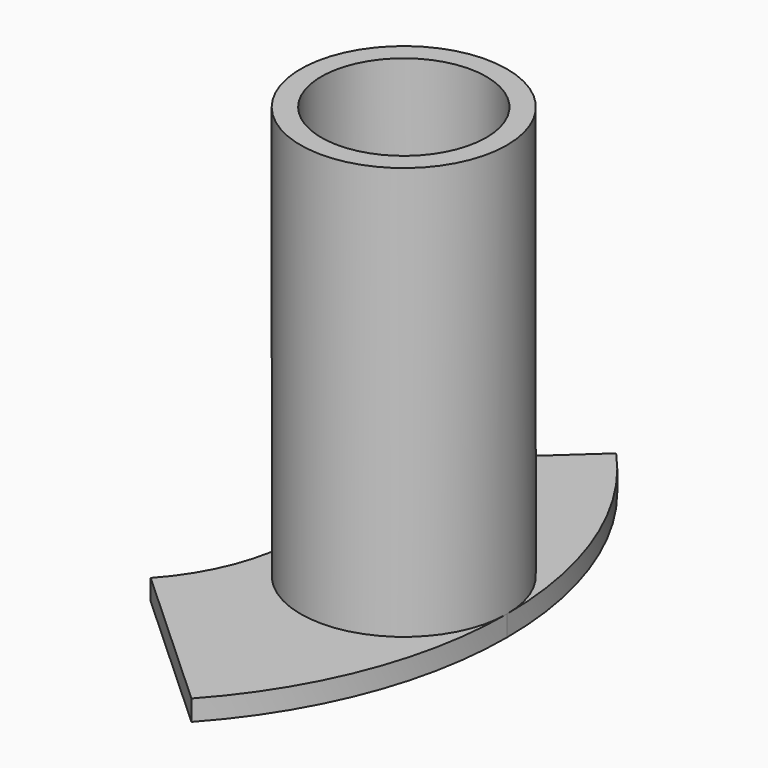
from build123d import *

# Parameters (mm, degrees)
F0_R     = 10
F1_DEPTH = 40
F2_R     = 8
F3_DEPTH = 35
F5_DEPTH = 2


with BuildPart() as f1:
    # F0 (on Top) → F1 (new body)
    with BuildSketch(Plane.XY):
        Circle(F0_R)
    extrude(amount=F1_DEPTH)

    # F2 (on face) → F3 (cut)
    with BuildSketch(Plane.XY.offset(40)):
        Circle(F2_R)
    extrude(amount=-F3_DEPTH, mode=Mode.SUBTRACT)

    # F4 (on face) → F5 (join)
    with BuildSketch(Plane(origin=(0, 0, 0), x_dir=(1, 0, 0), z_dir=(0, 0, -1))):
        with BuildLine():
            Line((-10, 0), (0, 0))
            Line((0, 0), (10, 0))
            ThreePointArc((10, 0), (0, 10), (-10, 0))
        make_face()
        with BuildLine():
            Line((10, 0), (0, 0))
            Line((0, 0), (-10, 0))
            ThreePointArc((-10, 0), (0, -10), (10, 0))
        make_face()
        with BuildLine():
            ThreePointArc((-10, 0), (0, 10), (10, 0))
            ThreePointArc((10, 0), (7.4121106103, 13.8021737418), (0, 25.7293606605))
            Line((0, 25.7293606605), (-14.750656168, 12.223134592))
            ThreePointArc((-14.750656168, 12.223134592), (-11.2294172691, 6.5569381818), (-10, 0))
        make_face()
        with BuildLine():
            ThreePointArc((0, -25.7293606605), (7.4121106103, -13.8021737418), (10, 0))
            ThreePointArc((10, 0), (0, -10), (-10, 0))
            ThreePointArc((-10, 0), (-11.2294172691, -6.5569381818), (-14.750656168, -12.223134592))
            Line((-14.750656168, -12.223134592), (0, -25.7293606605))
        make_face()
    extrude(amount=F5_DEPTH)


solid = f1.part
